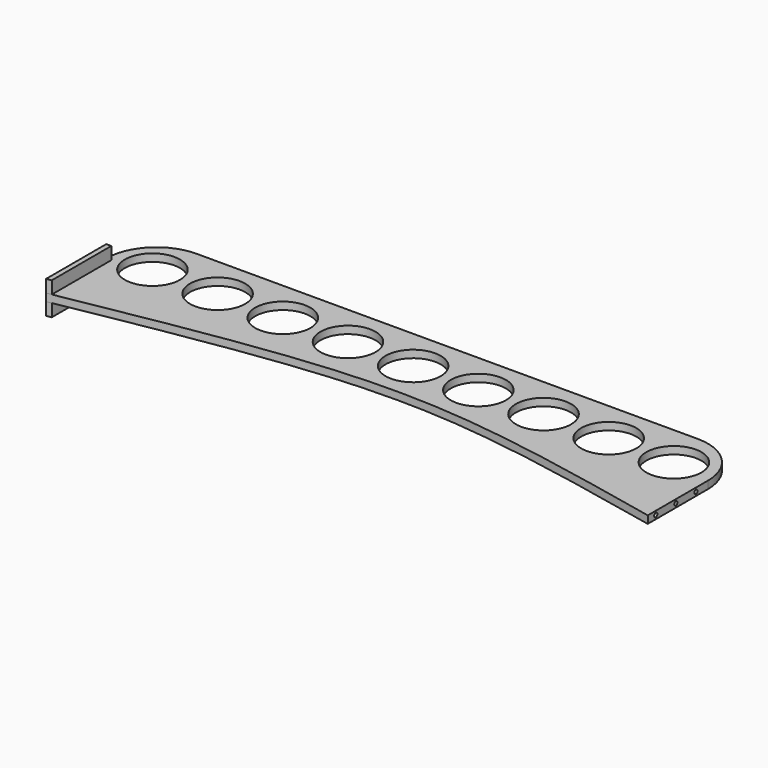
from build123d import *

# Parameters (mm, degrees)
F0_W      = 1200
F0_H      = 250
F1_DEPTH  = 15
F3_DEPTH  = 25
F4_R      = 100
F6_D      = 8
F6_DEPTH  = 60
F6_TIP    = 2.4034424761
F8_D      = 8
F8_DEPTH  = 60
F8_TIP    = 2.4034424761
F9_R      = 55
F10_DEPTH = 25
F12_DEPTH = 25
F14_DEPTH = 25


# Not quite as in the source:
# - a feature names something its author has since deleted; it is built from what else it names


with BuildPart() as f1:
    # F0 (on Top) → F1 (new body)
    with BuildSketch(Plane.XY):
        with Locations((-382.0752739906, 268.1212723255)):
            Rectangle(F0_W, F0_H)
    extrude(amount=F1_DEPTH)

    # F2 (on face) → F3 (cut)
    with BuildSketch(Plane.XY.offset(15)):
        with BuildLine():
            add(Edge.make_bspline(
                [(-982.0752739906, 143.1212723255), (-381.1290302773, 253.1212723255), (-296.0948119124, 253.1212723255), (217.9247260094, 143.1212723255)],
                knots=[0, 0, 0, 0, 1200, 1200, 1200, 1200], degree=3))
            Line((-982.0752739906, 143.1212723255), (217.9247260094, 143.1212723255))
        make_face()
    extrude(amount=-F3_DEPTH, mode=Mode.SUBTRACT)

    # F4
    f4_edges = [f1.edges().sort_by_distance(p)[0] for p in [
        (-982.075274, 393.121272, 7.5),
        (217.924726, 393.121272, 7.5),
    ]]
    fillet(f4_edges, radius=F4_R)

    # F6
    with Locations(Plane(origin=(-982.0752739906, 0, 0), x_dir=(0, -1, 0), z_dir=(-1, 0, 0))):
        with Locations((-163.1212723255, 7.5), (-213.1212723255, 7.5), (-263.1212723255, 7.5)):
            Hole(F6_D / 2, depth=F6_DEPTH)
            with Locations((0, 0, -(F6_DEPTH + F6_TIP / 2))):  # 118° drill point
                Cone(0, F6_D / 2, F6_TIP, mode=Mode.SUBTRACT)

    # F8
    with Locations(Plane.YZ.offset(217.9247260094)):
        with Locations((163.1212723255, 7.5), (213.1212723255, 7.5), (263.1212723255, 7.5)):
            Hole(F8_D / 2, depth=F8_DEPTH)
            with Locations((0, 0, -(F8_DEPTH + F8_TIP / 2))):  # 118° drill point
                Cone(0, F8_D / 2, F8_TIP, mode=Mode.SUBTRACT)

    # F9 (on face) → F10 (cut)
    with BuildSketch(Plane.XY.offset(15)):
        with Locations((-902.0752739906, 308.2580530366)):
            Circle(F9_R)
        with Locations((-772.0752739906, 308.2580530366)):
            Circle(F9_R)
        with Locations((-642.0752739906, 308.2580530366)):
            Circle(F9_R)
        with Locations((-512.0752739906, 308.2580530366)):
            Circle(F9_R)
        with Locations((-382.0752739906, 308.2580530366)):
            Circle(F9_R)
        with Locations((-252.0752739906, 308.2580530366)):
            Circle(F9_R)
        with Locations((-122.0752739906, 308.2580530366)):
            Circle(F9_R)
        with Locations((7.9247260094, 308.2580530366)):
            Circle(F9_R)
        with Locations((137.9247260094, 308.2580530366)):
            Circle(F9_R)
    extrude(amount=-F10_DEPTH, mode=Mode.SUBTRACT)

    # F11 (on face) → F12 (join)
    with BuildSketch(Plane(origin=(0, 0, 0), x_dir=(1, 0, 0), z_dir=(0, 0, -1))):
        with BuildLine():
            add(Edge.make_bspline(
                [(-972.0752739906, -144.9502384932), (-973.3234960268, -144.7221332236), (-974.5722289185, -144.4938787017), (-975.8214712324, -144.265475917), (-977.0712215354, -144.0369258537), (-978.3214783948, -143.8082294911), (-979.5722403783, -143.5793878034), (-980.823506054, -143.3504017601), (-982.0752739906, -143.1212723255)],
                knots=[0.9928997665, 0.9928997665, 0.9928997665, 0.9928997665, 0.9928997665, 0.9928997665, 0.9928997665, 0.9928997665, 0.9928997665, 1, 1, 1, 1, 1, 1, 1, 1, 1], degree=8))
            Line((-982.0752739906, -143.1212723255), (-982.0752739906, -293.1212723255))
            Line((-982.0752739906, -293.1212723255), (-972.0752739906, -293.1212723255))
            Line((-972.0752739906, -293.1212723255), (-972.0752739906, -144.9502384932))
        make_face()
    extrude(amount=F12_DEPTH)

    # F13 (on face) → F14 (join)
    with BuildSketch(Plane.XY.offset(15)):
        with BuildLine():
            Line((-982.0752739906, 293.1212723255), (-982.0752739906, 143.1212723255))
            add(Edge.make_bspline(
                [(-982.0752739906, 143.1212723255), (-978.7259696098, 143.7343446023), (-975.3926908046, 144.3439999918), (-972.0752739906, 144.9502384937)],
                knots=[0, 0, 0, 0, 6.6880612018, 6.6880612018, 6.6880612018, 6.6880612018], degree=3))
            Line((-972.0752739906, 144.9502384937), (-972.0752739906, 293.1212723255))
            Line((-972.0752739906, 293.1212723255), (-982.0752739906, 293.1212723255))
        make_face()
    extrude(amount=F14_DEPTH)


solid = f1.part
